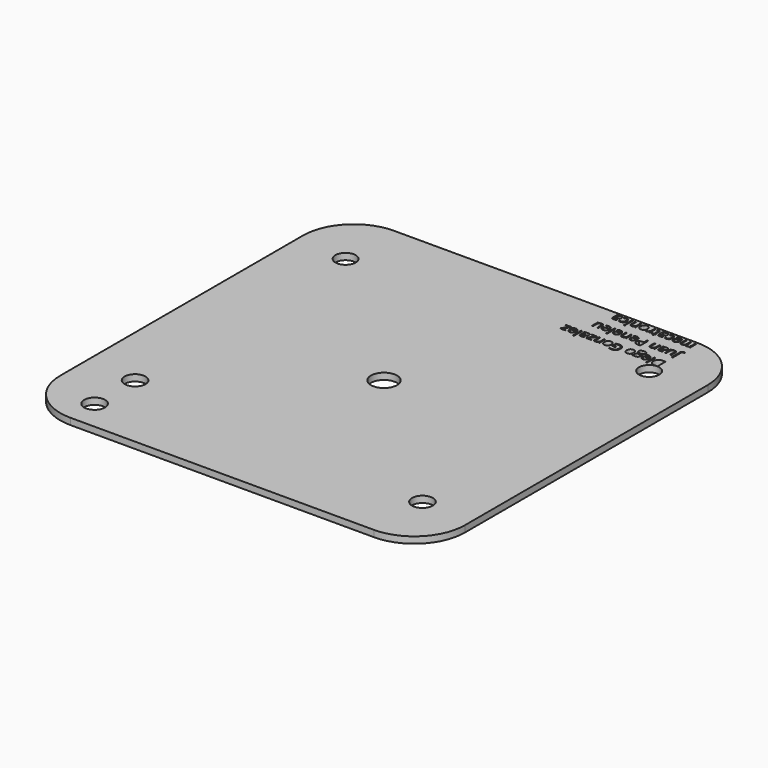
from build123d import *

# Parameters (mm, degrees)
F0_R     = 5.15
F0_R_2   = 5
F0_R_3   = 6.45
F0_W     = 0.5631510417
F0_H     = 5.2766927083
F0_H_2   = 3.7163628472
F1_DEPTH = 3.2


with BuildPart() as f1:
    # F0 (on Top) → F1 (new body)
    with BuildSketch(Plane.XY):
        with BuildLine():
            Line((75, 100), (-75, 100))
            ThreePointArc((-75, 100), (-92.6776695297, 92.6776695297), (-100, 75))
            Line((-100, 75), (-100, -75))
            ThreePointArc((-100, -75), (-92.6776695297, -92.6776695297), (-75, -100))
            Line((-75, -100), (75, -100))
            ThreePointArc((75, -100), (92.6776695297, -92.6776695297), (100, -75))
            Line((100, -75), (100, 75))
            ThreePointArc((100, 75), (92.6776695297, 92.6776695297), (75, 100))
        make_face()
        with Locations((-75, -85)):
            Circle(F0_R, mode=Mode.SUBTRACT)
        with Locations((-75, -60)):
            Circle(F0_R, mode=Mode.SUBTRACT)
        with Locations((75, -70)):
            Circle(F0_R, mode=Mode.SUBTRACT)
        with Locations((-75, 70)):
            Circle(F0_R_2, mode=Mode.SUBTRACT)
        Circle(F0_R_3, mode=Mode.SUBTRACT)
        Polygon((25.9928385417, 79.5627170139), (25.9928385417, 80), (28.6892361111, 80), (28.6892361111, 79.6169704861), (26.6612413194, 76.7209201389), (28.5633680556, 76.7209201389), (28.5633680556, 76.2836371528), (26.0438368056, 76.2836371528), (26.0438368056, 76.7209201389), (28.0447048611, 79.5627170139), align=None, mode=Mode.SUBTRACT)
        with BuildLine():
            add(Edge.make_bspline(
                [(30.0542534722, 80.0119357639), (30.3200954861, 80.068359375), (30.6966145833, 80.068359375)],
                knots=[0, 0, 0, 1, 1, 1], degree=2))
            add(Edge.make_bspline(
                [(30.6966145833, 80.068359375), (31.5201822917, 80.068359375), (31.9970703125, 79.5659722222)],
                knots=[0, 0, 0, 1, 1, 1], degree=2))
            add(Edge.make_bspline(
                [(31.9970703125, 79.5659722222), (32.4739583333, 79.0635850694), (32.4739583333, 78.1727430556)],
                knots=[0, 0, 0, 1, 1, 1], degree=2))
            add(Edge.make_bspline(
                [(32.4739583333, 78.1727430556), (32.4739583333, 77.2732204861), (32.03125, 76.7442491319)],
                knots=[0, 0, 0, 1, 1, 1], degree=2))
            add(Edge.make_bspline(
                [(32.03125, 76.7442491319), (31.5885416667, 76.2152777778), (30.8420138889, 76.2152777778)],
                knots=[0, 0, 0, 1, 1, 1], degree=2))
            add(Edge.make_bspline(
                [(30.8420138889, 76.2152777778), (30.1443142361, 76.2152777778), (29.7374131944, 76.6748046875)],
                knots=[0, 0, 0, 1, 1, 1], degree=2))
            add(Edge.make_bspline(
                [(29.7374131944, 76.6748046875), (29.3305121528, 77.1343315972), (29.3305121528, 77.8873697917)],
                knots=[0, 0, 0, 1, 1, 1], degree=2))
            Line((29.3305121528, 77.8873697917), (29.3305121528, 78.2432725694))
            Line((29.3305121528, 78.2432725694), (31.8901909722, 78.2432725694))
            add(Edge.make_bspline(
                [(31.8901909722, 78.2432725694), (31.8728298611, 78.8975694444), (31.5592447917, 79.2366536458)],
                knots=[0, 0, 0, 1, 1, 1], degree=2))
            add(Edge.make_bspline(
                [(31.5592447917, 79.2366536458), (31.2456597222, 79.5757378472), (30.6759982639, 79.5757378472)],
                knots=[0, 0, 0, 1, 1, 1], degree=2))
            add(Edge.make_bspline(
                [(30.6759982639, 79.5757378472), (30.0759548611, 79.5757378472), (29.4900173611, 79.3250868056)],
                knots=[0, 0, 0, 1, 1, 1], degree=2))
            Line((29.4900173611, 79.3250868056), (29.4900173611, 79.8274739583))
            add(Edge.make_bspline(
                [(29.4900173611, 79.8274739583), (29.7884114583, 79.9555121528), (30.0542534722, 80.0119357639)],
                knots=[0, 0, 0, 1, 1, 1], degree=2))
        make_face(mode=Mode.SUBTRACT)
        with Locations((33.7418619792, 77.3616536458)):
            Rectangle(F0_W, F0_H, mode=Mode.SUBTRACT)
        with BuildLine():
            Line((35.1822916667, 80), (35.6000434028, 80))
            Line((35.6000434028, 80), (35.7118055556, 79.4704861111))
            Line((35.7118055556, 79.4704861111), (35.7389322917, 79.4704861111))
            add(Edge.make_bspline(
                [(35.7389322917, 79.4704861111), (36.0167100694, 79.8198784722), (36.2928602431, 79.9441189236)],
                knots=[0, 0, 0, 1, 1, 1], degree=2))
            add(Edge.make_bspline(
                [(36.2928602431, 79.9441189236), (36.5690104167, 80.068359375), (36.9835069444, 80.068359375)],
                knots=[0, 0, 0, 1, 1, 1], degree=2))
            add(Edge.make_bspline(
                [(36.9835069444, 80.068359375), (37.5358072917, 80.068359375), (37.8493923611, 79.7829861111)],
                knots=[0, 0, 0, 1, 1, 1], degree=2))
            add(Edge.make_bspline(
                [(37.8493923611, 79.7829861111), (38.1629774306, 79.4976128472), (38.1629774306, 78.9724392361)],
                knots=[0, 0, 0, 1, 1, 1], degree=2))
            add(Edge.make_bspline(
                [(38.1629774306, 78.9724392361), (38.1629774306, 77.8472222222), (36.3628472222, 77.79296875)],
                knots=[0, 0, 0, 1, 1, 1], degree=2))
            Line((36.3628472222, 77.79296875), (35.732421875, 77.7723524306))
            Line((35.732421875, 77.7723524306), (35.732421875, 77.5412326389))
            add(Edge.make_bspline(
                [(35.732421875, 77.5412326389), (35.732421875, 77.1039496528), (35.9201388889, 76.8956163194)],
                knots=[0, 0, 0, 1, 1, 1], degree=2))
            add(Edge.make_bspline(
                [(35.9201388889, 76.8956163194), (36.1078559028, 76.6872829861), (36.5223524306, 76.6872829861)],
                knots=[0, 0, 0, 1, 1, 1], degree=2))
            add(Edge.make_bspline(
                [(36.5223524306, 76.6872829861), (36.9867621528, 76.6872829861), (37.5726996528, 76.9715711806)],
                knots=[0, 0, 0, 1, 1, 1], degree=2))
            Line((37.5726996528, 76.9715711806), (37.7463107639, 76.5407986111))
            add(Edge.make_bspline(
                [(37.7463107639, 76.5407986111), (37.4717881944, 76.3921440972), (37.1446397569, 76.3075086806)],
                knots=[0, 0, 0, 1, 1, 1], degree=2))
            add(Edge.make_bspline(
                [(37.1446397569, 76.3075086806), (36.8174913194, 76.2228732639), (36.4876302083, 76.2228732639)],
                knots=[0, 0, 0, 1, 1, 1], degree=2))
            add(Edge.make_bspline(
                [(36.4876302083, 76.2228732639), (35.8235677083, 76.2228732639), (35.5029296875, 76.5174696181)],
                knots=[0, 0, 0, 1, 1, 1], degree=2))
            add(Edge.make_bspline(
                [(35.5029296875, 76.5174696181), (35.1822916667, 76.8120659722), (35.1822916667, 77.4631076389)],
                knots=[0, 0, 0, 1, 1, 1], degree=2))
            Line((35.1822916667, 77.4631076389), (35.1822916667, 80))
        make_face(mode=Mode.SUBTRACT)
        Polygon((38.7565104167, 79.5627170139), (38.7565104167, 80), (41.4529079861, 80), (41.4529079861, 79.6169704861), (39.4249131944, 76.7209201389), (41.3270399306, 76.7209201389), (41.3270399306, 76.2836371528), (38.8075086806, 76.2836371528), (38.8075086806, 76.7209201389), (40.8083767361, 79.5627170139), align=None, mode=Mode.SUBTRACT)
        with BuildLine():
            Line((42.2894965278, 80), (42.8526475694, 80))
            Line((42.8526475694, 80), (42.8526475694, 77.5954861111))
            add(Edge.make_bspline(
                [(42.8526475694, 77.5954861111), (42.8526475694, 77.1419270833), (43.0593532986, 76.9178602431)],
                knots=[0, 0, 0, 1, 1, 1], degree=2))
            add(Edge.make_bspline(
                [(43.0593532986, 76.9178602431), (43.2660590278, 76.6937934028), (43.7076822917, 76.6937934028)],
                knots=[0, 0, 0, 1, 1, 1], degree=2))
            add(Edge.make_bspline(
                [(43.7076822917, 76.6937934028), (44.2903645833, 76.6937934028), (44.5616319444, 77.0090060764)],
                knots=[0, 0, 0, 1, 1, 1], degree=2))
            add(Edge.make_bspline(
                [(44.5616319444, 77.0090060764), (44.8328993056, 77.32421875), (44.8328993056, 78.0501302083)],
                knots=[0, 0, 0, 1, 1, 1], degree=2))
            Line((44.8328993056, 78.0501302083), (44.8328993056, 80))
            Line((44.8328993056, 80), (45.3960503472, 80))
            Line((45.3960503472, 80), (45.3960503472, 76.2836371528))
            Line((45.3960503472, 76.2836371528), (44.9381510417, 76.2836371528))
            Line((44.9381510417, 76.2836371528), (44.8470052083, 76.7925347222))
            Line((44.8470052083, 76.7925347222), (44.8198784722, 76.7925347222))
            add(Edge.make_bspline(
                [(44.8198784722, 76.7925347222), (44.6462673611, 76.5180121528), (44.3343098958, 76.3666449653)],
                knots=[0, 0, 0, 1, 1, 1], degree=2))
            add(Edge.make_bspline(
                [(44.3343098958, 76.3666449653), (44.0223524306, 76.2152777778), (43.6393229167, 76.2152777778)],
                knots=[0, 0, 0, 1, 1, 1], degree=2))
            add(Edge.make_bspline(
                [(43.6393229167, 76.2152777778), (42.9676649306, 76.2152777778), (42.6285807292, 76.5391710069)],
                knots=[0, 0, 0, 1, 1, 1], degree=2))
            add(Edge.make_bspline(
                [(42.6285807292, 76.5391710069), (42.2894965278, 76.8630642361), (42.2894965278, 77.5759548611)],
                knots=[0, 0, 0, 1, 1, 1], degree=2))
            Line((42.2894965278, 77.5759548611), (42.2894965278, 80))
        make_face(mode=Mode.SUBTRACT)
        with BuildLine():
            add(Edge.make_bspline(
                [(46.8429904514, 76.7344835069), (46.3834635417, 77.2536892361), (46.3834635417, 78.1380208333)],
                knots=[0, 0, 0, 1, 1, 1], degree=2))
            add(Edge.make_bspline(
                [(46.3834635417, 78.1380208333), (46.3834635417, 79.0473090278), (46.8408203125, 79.5578342014)],
                knots=[0, 0, 0, 1, 1, 1], degree=2))
            add(Edge.make_bspline(
                [(46.8408203125, 79.5578342014), (47.2981770833, 80.068359375), (48.10546875, 80.068359375)],
                knots=[0, 0, 0, 1, 1, 1], degree=2))
            add(Edge.make_bspline(
                [(48.10546875, 80.068359375), (48.6046006944, 80.068359375), (48.9908854167, 79.833984375)],
                knots=[0, 0, 0, 1, 1, 1], degree=2))
            add(Edge.make_bspline(
                [(48.9908854167, 79.833984375), (49.3771701389, 79.599609375), (49.5876736111, 79.1623263889)],
                knots=[0, 0, 0, 1, 1, 1], degree=2))
            add(Edge.make_bspline(
                [(49.5876736111, 79.1623263889), (49.7981770833, 78.7250434028), (49.7981770833, 78.1380208333)],
                knots=[0, 0, 0, 1, 1, 1], degree=2))
            add(Edge.make_bspline(
                [(49.7981770833, 78.1380208333), (49.7981770833, 77.2298177083), (49.3435329861, 76.7225477431)],
                knots=[0, 0, 0, 1, 1, 1], degree=2))
            add(Edge.make_bspline(
                [(49.3435329861, 76.7225477431), (48.8888888889, 76.2152777778), (48.0815972222, 76.2152777778)],
                knots=[0, 0, 0, 1, 1, 1], degree=2))
            add(Edge.make_bspline(
                [(48.0815972222, 76.2152777778), (47.3025173611, 76.2152777778), (46.8429904514, 76.7344835069)],
                knots=[0, 0, 0, 1, 1, 1], degree=2))
        make_face(mode=Mode.SUBTRACT)
        with Locations((42.6036241319, 86.8060980903)):
            Rectangle(F0_W, F0_H, mode=Mode.SUBTRACT)
        with BuildLine():
            Line((37.2721354167, 85.7280815972), (36.7024739583, 85.7280815972))
            Line((36.7024739583, 85.7280815972), (36.7024739583, 88.1391059028))
            add(Edge.make_bspline(
                [(36.7024739583, 88.1391059028), (36.7024739583, 88.59375), (36.4957682292, 88.8172743056)],
                knots=[0, 0, 0, 1, 1, 1], degree=2))
            add(Edge.make_bspline(
                [(36.4957682292, 88.8172743056), (36.2890625, 89.0407986111), (35.8485243056, 89.0407986111)],
                knots=[0, 0, 0, 1, 1, 1], degree=2))
            add(Edge.make_bspline(
                [(35.8485243056, 89.0407986111), (35.2647569444, 89.0407986111), (34.9956597222, 88.7223307292)],
                knots=[0, 0, 0, 1, 1, 1], degree=2))
            add(Edge.make_bspline(
                [(34.9956597222, 88.7223307292), (34.7265625, 88.4038628472), (34.7265625, 87.6812065972)],
                knots=[0, 0, 0, 1, 1, 1], degree=2))
            Line((34.7265625, 87.6812065972), (34.7265625, 85.7280815972))
            Line((34.7265625, 85.7280815972), (34.1634114583, 85.7280815972))
            Line((34.1634114583, 85.7280815972), (34.1634114583, 89.4444444444))
            Line((34.1634114583, 89.4444444444), (34.6278211806, 89.4444444444))
            Line((34.6278211806, 89.4444444444), (34.7092013889, 88.9463975694))
            Line((34.7092013889, 88.9463975694), (34.7395833333, 88.9463975694))
            add(Edge.make_bspline(
                [(34.7395833333, 88.9463975694), (34.912109375, 89.2209201389), (35.2191840278, 89.3668619792)],
                knots=[0, 0, 0, 1, 1, 1], degree=2))
            add(Edge.make_bspline(
                [(35.2191840278, 89.3668619792), (35.5262586806, 89.5128038194), (35.9201388889, 89.5128038194)],
                knots=[0, 0, 0, 1, 1, 1], degree=2))
            add(Edge.make_bspline(
                [(35.9201388889, 89.5128038194), (36.5983072917, 89.5128038194), (36.9352213542, 89.1905381944)],
                knots=[0, 0, 0, 1, 1, 1], degree=2))
            add(Edge.make_bspline(
                [(36.9352213542, 89.1905381944), (37.2721354167, 88.8682725694), (37.2721354167, 88.1597222222)],
                knots=[0, 0, 0, 1, 1, 1], degree=2))
            Line((37.2721354167, 88.1597222222), (37.2721354167, 85.7280815972))
        make_face(mode=Mode.SUBTRACT)
        with BuildLine():
            add(Edge.make_bspline(
                [(38.916015625, 89.4563802083), (39.1818576389, 89.5128038194), (39.5583767361, 89.5128038194)],
                knots=[0, 0, 0, 1, 1, 1], degree=2))
            add(Edge.make_bspline(
                [(39.5583767361, 89.5128038194), (40.3819444444, 89.5128038194), (40.8588324653, 89.0104166667)],
                knots=[0, 0, 0, 1, 1, 1], degree=2))
            add(Edge.make_bspline(
                [(40.8588324653, 89.0104166667), (41.3357204861, 88.5080295139), (41.3357204861, 87.6171875)],
                knots=[0, 0, 0, 1, 1, 1], degree=2))
            add(Edge.make_bspline(
                [(41.3357204861, 87.6171875), (41.3357204861, 86.7176649306), (40.8930121528, 86.1886935764)],
                knots=[0, 0, 0, 1, 1, 1], degree=2))
            add(Edge.make_bspline(
                [(40.8930121528, 86.1886935764), (40.4503038194, 85.6597222222), (39.7037760417, 85.6597222222)],
                knots=[0, 0, 0, 1, 1, 1], degree=2))
            add(Edge.make_bspline(
                [(39.7037760417, 85.6597222222), (39.0060763889, 85.6597222222), (38.5991753472, 86.1192491319)],
                knots=[0, 0, 0, 1, 1, 1], degree=2))
            add(Edge.make_bspline(
                [(38.5991753472, 86.1192491319), (38.1922743056, 86.5787760417), (38.1922743056, 87.3318142361)],
                knots=[0, 0, 0, 1, 1, 1], degree=2))
            Line((38.1922743056, 87.3318142361), (38.1922743056, 87.6877170139))
            Line((38.1922743056, 87.6877170139), (40.751953125, 87.6877170139))
            add(Edge.make_bspline(
                [(40.751953125, 87.6877170139), (40.7345920139, 88.3420138889), (40.4210069444, 88.6810980903)],
                knots=[0, 0, 0, 1, 1, 1], degree=2))
            add(Edge.make_bspline(
                [(40.4210069444, 88.6810980903), (40.107421875, 89.0201822917), (39.5377604167, 89.0201822917)],
                knots=[0, 0, 0, 1, 1, 1], degree=2))
            add(Edge.make_bspline(
                [(39.5377604167, 89.0201822917), (38.9377170139, 89.0201822917), (38.3517795139, 88.76953125)],
                knots=[0, 0, 0, 1, 1, 1], degree=2))
            Line((38.3517795139, 88.76953125), (38.3517795139, 89.2719184028))
            add(Edge.make_bspline(
                [(38.3517795139, 89.2719184028), (38.6501736111, 89.3999565972), (38.916015625, 89.4563802083)],
                knots=[0, 0, 0, 1, 1, 1], degree=2))
        make_face(mode=Mode.SUBTRACT)
        with BuildLine():
            add(Edge.make_bspline(
                [(44.5692274306, 89.4563802083), (44.8350694444, 89.5128038194), (45.2115885417, 89.5128038194)],
                knots=[0, 0, 0, 1, 1, 1], degree=2))
            add(Edge.make_bspline(
                [(45.2115885417, 89.5128038194), (46.03515625, 89.5128038194), (46.5120442708, 89.0104166667)],
                knots=[0, 0, 0, 1, 1, 1], degree=2))
            add(Edge.make_bspline(
                [(46.5120442708, 89.0104166667), (46.9889322917, 88.5080295139), (46.9889322917, 87.6171875)],
                knots=[0, 0, 0, 1, 1, 1], degree=2))
            add(Edge.make_bspline(
                [(46.9889322917, 87.6171875), (46.9889322917, 86.7176649306), (46.5462239583, 86.1886935764)],
                knots=[0, 0, 0, 1, 1, 1], degree=2))
            add(Edge.make_bspline(
                [(46.5462239583, 86.1886935764), (46.103515625, 85.6597222222), (45.3569878472, 85.6597222222)],
                knots=[0, 0, 0, 1, 1, 1], degree=2))
            add(Edge.make_bspline(
                [(45.3569878472, 85.6597222222), (44.6592881944, 85.6597222222), (44.2523871528, 86.1192491319)],
                knots=[0, 0, 0, 1, 1, 1], degree=2))
            add(Edge.make_bspline(
                [(44.2523871528, 86.1192491319), (43.8454861111, 86.5787760417), (43.8454861111, 87.3318142361)],
                knots=[0, 0, 0, 1, 1, 1], degree=2))
            Line((43.8454861111, 87.3318142361), (43.8454861111, 87.6877170139))
            Line((43.8454861111, 87.6877170139), (46.4051649306, 87.6877170139))
            add(Edge.make_bspline(
                [(46.4051649306, 87.6877170139), (46.3878038194, 88.3420138889), (46.07421875, 88.6810980903)],
                knots=[0, 0, 0, 1, 1, 1], degree=2))
            add(Edge.make_bspline(
                [(46.07421875, 88.6810980903), (45.7606336806, 89.0201822917), (45.1909722222, 89.0201822917)],
                knots=[0, 0, 0, 1, 1, 1], degree=2))
            add(Edge.make_bspline(
                [(45.1909722222, 89.0201822917), (44.5909288194, 89.0201822917), (44.0049913194, 88.76953125)],
                knots=[0, 0, 0, 1, 1, 1], degree=2))
            Line((44.0049913194, 88.76953125), (44.0049913194, 89.2719184028))
            add(Edge.make_bspline(
                [(44.0049913194, 89.2719184028), (44.3033854167, 89.3999565972), (44.5692274306, 89.4563802083)],
                knots=[0, 0, 0, 1, 1, 1], degree=2))
        make_face(mode=Mode.SUBTRACT)
        with BuildLine():
            Line((47.9372829861, 89.4444444444), (48.5004340278, 89.4444444444))
            Line((48.5004340278, 89.4444444444), (48.5004340278, 87.0399305556))
            add(Edge.make_bspline(
                [(48.5004340278, 87.0399305556), (48.5004340278, 86.5863715278), (48.7071397569, 86.3623046875)],
                knots=[0, 0, 0, 1, 1, 1], degree=2))
            add(Edge.make_bspline(
                [(48.7071397569, 86.3623046875), (48.9138454861, 86.1382378472), (49.35546875, 86.1382378472)],
                knots=[0, 0, 0, 1, 1, 1], degree=2))
            add(Edge.make_bspline(
                [(49.35546875, 86.1382378472), (49.9381510417, 86.1382378472), (50.2094184028, 86.4534505208)],
                knots=[0, 0, 0, 1, 1, 1], degree=2))
            add(Edge.make_bspline(
                [(50.2094184028, 86.4534505208), (50.4806857639, 86.7686631944), (50.4806857639, 87.4945746528)],
                knots=[0, 0, 0, 1, 1, 1], degree=2))
            Line((50.4806857639, 87.4945746528), (50.4806857639, 89.4444444444))
            Line((50.4806857639, 89.4444444444), (51.0438368056, 89.4444444444))
            Line((51.0438368056, 89.4444444444), (51.0438368056, 85.7280815972))
            Line((51.0438368056, 85.7280815972), (50.5859375, 85.7280815972))
            Line((50.5859375, 85.7280815972), (50.4947916667, 86.2369791667))
            Line((50.4947916667, 86.2369791667), (50.4676649306, 86.2369791667))
            add(Edge.make_bspline(
                [(50.4676649306, 86.2369791667), (50.2940538194, 85.9624565972), (49.9820963542, 85.8110894097)],
                knots=[0, 0, 0, 1, 1, 1], degree=2))
            add(Edge.make_bspline(
                [(49.9820963542, 85.8110894097), (49.6701388889, 85.6597222222), (49.287109375, 85.6597222222)],
                knots=[0, 0, 0, 1, 1, 1], degree=2))
            add(Edge.make_bspline(
                [(49.287109375, 85.6597222222), (48.6154513889, 85.6597222222), (48.2763671875, 85.9836154514)],
                knots=[0, 0, 0, 1, 1, 1], degree=2))
            add(Edge.make_bspline(
                [(48.2763671875, 85.9836154514), (47.9372829861, 86.3075086806), (47.9372829861, 87.0203993056)],
                knots=[0, 0, 0, 1, 1, 1], degree=2))
            Line((47.9372829861, 87.0203993056), (47.9372829861, 89.4444444444))
        make_face(mode=Mode.SUBTRACT)
        with BuildLine():
            add(Edge.make_bspline(
                [(43.8514539931, 94.4487847222), (43.9463975694, 94.35546875), (43.9463975694, 94.1655815972)],
                knots=[0, 0, 0, 1, 1, 1], degree=2))
            add(Edge.make_bspline(
                [(43.9463975694, 94.1655815972), (43.9463975694, 93.9724392361), (43.8514539931, 93.8823784722)],
                knots=[0, 0, 0, 1, 1, 1], degree=2))
            add(Edge.make_bspline(
                [(43.8514539931, 93.8823784722), (43.7565104167, 93.7923177083), (43.61328125, 93.7923177083)],
                knots=[0, 0, 0, 1, 1, 1], degree=2))
            add(Edge.make_bspline(
                [(43.61328125, 93.7923177083), (43.4776475694, 93.7923177083), (43.3794487847, 93.8840060764)],
                knots=[0, 0, 0, 1, 1, 1], degree=2))
            add(Edge.make_bspline(
                [(43.3794487847, 93.8840060764), (43.28125, 93.9756944444), (43.28125, 94.1655815972)],
                knots=[0, 0, 0, 1, 1, 1], degree=2))
            add(Edge.make_bspline(
                [(43.28125, 94.1655815972), (43.28125, 94.35546875), (43.3794487847, 94.4487847222)],
                knots=[0, 0, 0, 1, 1, 1], degree=2))
            add(Edge.make_bspline(
                [(43.3794487847, 94.4487847222), (43.4776475694, 94.5421006944), (43.61328125, 94.5421006944)],
                knots=[0, 0, 0, 1, 1, 1], degree=2))
            add(Edge.make_bspline(
                [(43.61328125, 94.5421006944), (43.7565104167, 94.5421006944), (43.8514539931, 94.4487847222)],
                knots=[0, 0, 0, 1, 1, 1], degree=2))
        make_face(mode=Mode.SUBTRACT)
        with BuildLine():
            Line((36.1328125, 98.8888888889), (36.5505642361, 98.8888888889))
            Line((36.5505642361, 98.8888888889), (36.6623263889, 98.359375))
            Line((36.6623263889, 98.359375), (36.689453125, 98.359375))
            add(Edge.make_bspline(
                [(36.689453125, 98.359375), (36.9672309028, 98.7087673611), (37.2433810764, 98.8330078125)],
                knots=[0, 0, 0, 1, 1, 1], degree=2))
            add(Edge.make_bspline(
                [(37.2433810764, 98.8330078125), (37.51953125, 98.9572482639), (37.9340277778, 98.9572482639)],
                knots=[0, 0, 0, 1, 1, 1], degree=2))
            add(Edge.make_bspline(
                [(37.9340277778, 98.9572482639), (38.486328125, 98.9572482639), (38.7999131944, 98.671875)],
                knots=[0, 0, 0, 1, 1, 1], degree=2))
            add(Edge.make_bspline(
                [(38.7999131944, 98.671875), (39.1134982639, 98.3865017361), (39.1134982639, 97.861328125)],
                knots=[0, 0, 0, 1, 1, 1], degree=2))
            add(Edge.make_bspline(
                [(39.1134982639, 97.861328125), (39.1134982639, 96.7361111111), (37.3133680556, 96.6818576389)],
                knots=[0, 0, 0, 1, 1, 1], degree=2))
            Line((37.3133680556, 96.6818576389), (36.6829427083, 96.6612413194))
            Line((36.6829427083, 96.6612413194), (36.6829427083, 96.4301215278))
            add(Edge.make_bspline(
                [(36.6829427083, 96.4301215278), (36.6829427083, 95.9928385417), (36.8706597222, 95.7845052083)],
                knots=[0, 0, 0, 1, 1, 1], degree=2))
            add(Edge.make_bspline(
                [(36.8706597222, 95.7845052083), (37.0583767361, 95.576171875), (37.4728732639, 95.576171875)],
                knots=[0, 0, 0, 1, 1, 1], degree=2))
            add(Edge.make_bspline(
                [(37.4728732639, 95.576171875), (37.9372829861, 95.576171875), (38.5232204861, 95.8604600694)],
                knots=[0, 0, 0, 1, 1, 1], degree=2))
            Line((38.5232204861, 95.8604600694), (38.6968315972, 95.4296875))
            add(Edge.make_bspline(
                [(38.6968315972, 95.4296875), (38.4223090278, 95.2810329861), (38.0951605903, 95.1963975694)],
                knots=[0, 0, 0, 1, 1, 1], degree=2))
            add(Edge.make_bspline(
                [(38.0951605903, 95.1963975694), (37.7680121528, 95.1117621528), (37.4381510417, 95.1117621528)],
                knots=[0, 0, 0, 1, 1, 1], degree=2))
            add(Edge.make_bspline(
                [(37.4381510417, 95.1117621528), (36.7740885417, 95.1117621528), (36.4534505208, 95.4063585069)],
                knots=[0, 0, 0, 1, 1, 1], degree=2))
            add(Edge.make_bspline(
                [(36.4534505208, 95.4063585069), (36.1328125, 95.7009548611), (36.1328125, 96.3519965278)],
                knots=[0, 0, 0, 1, 1, 1], degree=2))
            Line((36.1328125, 96.3519965278), (36.1328125, 98.8888888889))
        make_face(mode=Mode.SUBTRACT)
        with BuildLine():
            add(Edge.make_bspline(
                [(39.7178819444, 98.7630208333), (40.0900607639, 98.9572482639), (40.6564670139, 98.9572482639)],
                knots=[0, 0, 0, 1, 1, 1], degree=2))
            add(Edge.make_bspline(
                [(40.6564670139, 98.9572482639), (41.4637586806, 98.9572482639), (41.9064670139, 98.4602864583)],
                knots=[0, 0, 0, 1, 1, 1], degree=2))
            add(Edge.make_bspline(
                [(41.9064670139, 98.4602864583), (42.3491753472, 97.9633246528), (42.3491753472, 97.0540364583)],
                knots=[0, 0, 0, 1, 1, 1], degree=2))
            add(Edge.make_bspline(
                [(42.3491753472, 97.0540364583), (42.3491753472, 96.1219618056), (41.8994140625, 95.6130642361)],
                knots=[0, 0, 0, 1, 1, 1], degree=2))
            add(Edge.make_bspline(
                [(41.8994140625, 95.6130642361), (41.4496527778, 95.1041666667), (40.6195746528, 95.1041666667)],
                knots=[0, 0, 0, 1, 1, 1], degree=2))
            add(Edge.make_bspline(
                [(40.6195746528, 95.1041666667), (40.3515625, 95.1041666667), (40.0835503472, 95.1622178819)],
                knots=[0, 0, 0, 1, 1, 1], degree=2))
            add(Edge.make_bspline(
                [(40.0835503472, 95.1622178819), (39.8155381944, 95.2202690972), (39.6636284722, 95.2983940972)],
                knots=[0, 0, 0, 1, 1, 1], degree=2))
            Line((39.6636284722, 95.2983940972), (39.8361545139, 95.7758246528))
            add(Edge.make_bspline(
                [(39.8361545139, 95.7758246528), (40.0227864583, 95.7009548611), (40.2430555556, 95.6521267361)],
                knots=[0, 0, 0, 1, 1, 1], degree=2))
            add(Edge.make_bspline(
                [(40.2430555556, 95.6521267361), (40.4633246528, 95.6032986111), (40.6325954861, 95.6032986111)],
                knots=[0, 0, 0, 1, 1, 1], degree=2))
            add(Edge.make_bspline(
                [(40.6325954861, 95.6032986111), (41.7654079861, 95.6032986111), (41.7654079861, 97.0475260417)],
                knots=[0, 0, 0, 1, 1, 1], degree=2))
            add(Edge.make_bspline(
                [(41.7654079861, 97.0475260417), (41.7654079861, 97.7322048611), (41.4892578125, 98.0984157986)],
                knots=[0, 0, 0, 1, 1, 1], degree=2))
            add(Edge.make_bspline(
                [(41.4892578125, 98.0984157986), (41.2131076389, 98.4646267361), (40.6705729167, 98.4646267361)],
                knots=[0, 0, 0, 1, 1, 1], degree=2))
            add(Edge.make_bspline(
                [(40.6705729167, 98.4646267361), (40.2061631944, 98.4646267361), (39.7178819444, 98.2649739583)],
                knots=[0, 0, 0, 1, 1, 1], degree=2))
            Line((39.7178819444, 98.2649739583), (39.7178819444, 98.7630208333))
        make_face(mode=Mode.SUBTRACT)
        with Locations((43.6170789931, 97.0307074653)):
            Rectangle(F0_W, F0_H_2, mode=Mode.SUBTRACT)
        with BuildLine():
            Line((45.0542534722, 98.8888888889), (45.6174045139, 98.8888888889))
            Line((45.6174045139, 98.8888888889), (45.6174045139, 96.484375))
            add(Edge.make_bspline(
                [(45.6174045139, 96.484375), (45.6174045139, 96.0308159722), (45.8241102431, 95.8067491319)],
                knots=[0, 0, 0, 1, 1, 1], degree=2))
            add(Edge.make_bspline(
                [(45.8241102431, 95.8067491319), (46.0308159722, 95.5826822917), (46.4724392361, 95.5826822917)],
                knots=[0, 0, 0, 1, 1, 1], degree=2))
            add(Edge.make_bspline(
                [(46.4724392361, 95.5826822917), (47.0551215278, 95.5826822917), (47.3263888889, 95.8978949653)],
                knots=[0, 0, 0, 1, 1, 1], degree=2))
            add(Edge.make_bspline(
                [(47.3263888889, 95.8978949653), (47.59765625, 96.2131076389), (47.59765625, 96.9390190972)],
                knots=[0, 0, 0, 1, 1, 1], degree=2))
            Line((47.59765625, 96.9390190972), (47.59765625, 98.8888888889))
            Line((47.59765625, 98.8888888889), (48.1608072917, 98.8888888889))
            Line((48.1608072917, 98.8888888889), (48.1608072917, 95.1725260417))
            Line((48.1608072917, 95.1725260417), (47.7029079861, 95.1725260417))
            Line((47.7029079861, 95.1725260417), (47.6117621528, 95.6814236111))
            Line((47.6117621528, 95.6814236111), (47.5846354167, 95.6814236111))
            add(Edge.make_bspline(
                [(47.5846354167, 95.6814236111), (47.4110243056, 95.4069010417), (47.0990668403, 95.2555338542)],
                knots=[0, 0, 0, 1, 1, 1], degree=2))
            add(Edge.make_bspline(
                [(47.0990668403, 95.2555338542), (46.787109375, 95.1041666667), (46.4040798611, 95.1041666667)],
                knots=[0, 0, 0, 1, 1, 1], degree=2))
            add(Edge.make_bspline(
                [(46.4040798611, 95.1041666667), (45.732421875, 95.1041666667), (45.3933376736, 95.4280598958)],
                knots=[0, 0, 0, 1, 1, 1], degree=2))
            add(Edge.make_bspline(
                [(45.3933376736, 95.4280598958), (45.0542534722, 95.751953125), (45.0542534722, 96.46484375)],
                knots=[0, 0, 0, 1, 1, 1], degree=2))
            Line((45.0542534722, 96.46484375), (45.0542534722, 98.8888888889))
        make_face(mode=Mode.SUBTRACT)
        with Locations((75, 70)):
            Circle(F0_R_2, mode=Mode.SUBTRACT)
        with BuildLine():
            Line((52.3806423611, 77.9177517361), (52.3806423611, 77.40234375))
            Line((52.3806423611, 77.40234375), (50.6955295139, 77.40234375))
            Line((50.6955295139, 77.40234375), (50.6955295139, 79.8133680556))
            add(Edge.make_bspline(
                [(50.6955295139, 79.8133680556), (51.0894097222, 79.9392361111), (51.4963107639, 80.0037977431)],
                knots=[0, 0, 0, 1, 1, 1], degree=2))
            add(Edge.make_bspline(
                [(51.4963107639, 80.0037977431), (51.9032118056, 80.068359375), (52.4392361111, 80.068359375)],
                knots=[0, 0, 0, 1, 1, 1], degree=2))
            add(Edge.make_bspline(
                [(52.4392361111, 80.068359375), (53.564453125, 80.068359375), (54.1916232639, 79.3983289931)],
                knots=[0, 0, 0, 1, 1, 1], degree=2))
            add(Edge.make_bspline(
                [(54.1916232639, 79.3983289931), (54.8187934028, 78.7282986111), (54.8187934028, 77.5217013889)],
                knots=[0, 0, 0, 1, 1, 1], degree=2))
            add(Edge.make_bspline(
                [(54.8187934028, 77.5217013889), (54.8187934028, 76.748046875), (54.5084635417, 76.1664496528)],
                knots=[0, 0, 0, 1, 1, 1], degree=2))
            add(Edge.make_bspline(
                [(54.5084635417, 76.1664496528), (54.1981336806, 75.5848524306), (53.6149088542, 75.2783203125)],
                knots=[0, 0, 0, 1, 1, 1], degree=2))
            add(Edge.make_bspline(
                [(53.6149088542, 75.2783203125), (53.0316840278, 74.9717881944), (52.2493489583, 74.9717881944)],
                knots=[0, 0, 0, 1, 1, 1], degree=2))
            add(Edge.make_bspline(
                [(52.2493489583, 74.9717881944), (51.455078125, 74.9717881944), (50.7703993056, 75.2625868056)],
                knots=[0, 0, 0, 1, 1, 1], degree=2))
            Line((50.7703993056, 75.2625868056), (50.9939236111, 75.771484375))
            add(Edge.make_bspline(
                [(50.9939236111, 75.771484375), (51.6655815972, 75.4871961806), (52.2862413194, 75.4871961806)],
                knots=[0, 0, 0, 1, 1, 1], degree=2))
            add(Edge.make_bspline(
                [(52.2862413194, 75.4871961806), (53.1911892361, 75.4871961806), (53.7000868056, 76.0259331597)],
                knots=[0, 0, 0, 1, 1, 1], degree=2))
            add(Edge.make_bspline(
                [(53.7000868056, 76.0259331597), (54.208984375, 76.5646701389), (54.208984375, 77.5217013889)],
                knots=[0, 0, 0, 1, 1, 1], degree=2))
            add(Edge.make_bspline(
                [(54.208984375, 77.5217013889), (54.208984375, 78.525390625), (53.7190755208, 79.0440538194)],
                knots=[0, 0, 0, 1, 1, 1], degree=2))
            add(Edge.make_bspline(
                [(53.7190755208, 79.0440538194), (53.2291666667, 79.5627170139), (52.2797309028, 79.5627170139)],
                knots=[0, 0, 0, 1, 1, 1], degree=2))
            add(Edge.make_bspline(
                [(52.2797309028, 79.5627170139), (51.7643229167, 79.5627170139), (51.2727864583, 79.443359375)],
                knots=[0, 0, 0, 1, 1, 1], degree=2))
            Line((51.2727864583, 79.443359375), (51.2727864583, 77.9177517361))
            Line((51.2727864583, 77.9177517361), (52.3806423611, 77.9177517361))
        make_face(mode=Mode.SUBTRACT)
        with BuildLine():
            add(Edge.make_bspline(
                [(57.8976779514, 76.7344835069), (57.4381510417, 77.2536892361), (57.4381510417, 78.1380208333)],
                knots=[0, 0, 0, 1, 1, 1], degree=2))
            add(Edge.make_bspline(
                [(57.4381510417, 78.1380208333), (57.4381510417, 79.0473090278), (57.8955078125, 79.5578342014)],
                knots=[0, 0, 0, 1, 1, 1], degree=2))
            add(Edge.make_bspline(
                [(57.8955078125, 79.5578342014), (58.3528645833, 80.068359375), (59.16015625, 80.068359375)],
                knots=[0, 0, 0, 1, 1, 1], degree=2))
            add(Edge.make_bspline(
                [(59.16015625, 80.068359375), (59.6592881944, 80.068359375), (60.0455729167, 79.833984375)],
                knots=[0, 0, 0, 1, 1, 1], degree=2))
            add(Edge.make_bspline(
                [(60.0455729167, 79.833984375), (60.4318576389, 79.599609375), (60.6423611111, 79.1623263889)],
                knots=[0, 0, 0, 1, 1, 1], degree=2))
            add(Edge.make_bspline(
                [(60.6423611111, 79.1623263889), (60.8528645833, 78.7250434028), (60.8528645833, 78.1380208333)],
                knots=[0, 0, 0, 1, 1, 1], degree=2))
            add(Edge.make_bspline(
                [(60.8528645833, 78.1380208333), (60.8528645833, 77.2298177083), (60.3982204861, 76.7225477431)],
                knots=[0, 0, 0, 1, 1, 1], degree=2))
            add(Edge.make_bspline(
                [(60.3982204861, 76.7225477431), (59.9435763889, 76.2152777778), (59.1362847222, 76.2152777778)],
                knots=[0, 0, 0, 1, 1, 1], degree=2))
            add(Edge.make_bspline(
                [(59.1362847222, 76.2152777778), (58.3572048611, 76.2152777778), (57.8976779514, 76.7344835069)],
                knots=[0, 0, 0, 1, 1, 1], degree=2))
        make_face(mode=Mode.SUBTRACT)
        with BuildLine():
            add(Edge.make_bspline(
                [(57.7506510417, 84.4867621528), (55.8930121528, 84.4867621528), (55.8930121528, 85.9309895833)],
                knots=[0, 0, 0, 1, 1, 1], degree=2))
            add(Edge.make_bspline(
                [(55.8930121528, 85.9309895833), (55.8930121528, 86.6840277778), (56.4067925347, 87.0893012153)],
                knots=[0, 0, 0, 1, 1, 1], degree=2))
            add(Edge.make_bspline(
                [(56.4067925347, 87.0893012153), (56.9205729167, 87.4945746528), (57.8765190972, 87.4945746528)],
                knots=[0, 0, 0, 1, 1, 1], degree=2))
            Line((57.8765190972, 87.4945746528), (58.4602864583, 87.4945746528))
            Line((58.4602864583, 87.4945746528), (58.4602864583, 89.4444444444))
            Line((58.4602864583, 89.4444444444), (59.0364583333, 89.4444444444))
            Line((59.0364583333, 89.4444444444), (59.0364583333, 84.4867621528))
            Line((59.0364583333, 84.4867621528), (57.7506510417, 84.4867621528))
        make_face(mode=Mode.SUBTRACT)
        with BuildLine():
            Line((62.6931423611, 76.2836371528), (61.4084201389, 76.2836371528))
            Line((61.4084201389, 76.2836371528), (61.4084201389, 76.6395399306))
            Line((61.4084201389, 76.6395399306), (62.0963541667, 76.7209201389))
            add(Edge.make_bspline(
                [(62.0963541667, 76.7209201389), (62.001953125, 76.8391927083), (61.9270833333, 77.03125)],
                knots=[0, 0, 0, 1, 1, 1], degree=2))
            add(Edge.make_bspline(
                [(61.9270833333, 77.03125), (61.8522135417, 77.2233072917), (61.8522135417, 77.4631076389)],
                knots=[0, 0, 0, 1, 1, 1], degree=2))
            add(Edge.make_bspline(
                [(61.8522135417, 77.4631076389), (61.8522135417, 78.0099826389), (62.2254774306, 78.3355034722)],
                knots=[0, 0, 0, 1, 1, 1], degree=2))
            add(Edge.make_bspline(
                [(62.2254774306, 78.3355034722), (62.5987413194, 78.6610243056), (63.2497829861, 78.6610243056)],
                knots=[0, 0, 0, 1, 1, 1], degree=2))
            add(Edge.make_bspline(
                [(63.2497829861, 78.6610243056), (63.4157986111, 78.6610243056), (63.5611979167, 78.6338975694)],
                knots=[0, 0, 0, 1, 1, 1], degree=2))
            add(Edge.make_bspline(
                [(63.5611979167, 78.6338975694), (63.9203559028, 78.8237847222), (63.9203559028, 79.111328125)],
                knots=[0, 0, 0, 1, 1, 1], degree=2))
            add(Edge.make_bspline(
                [(63.9203559028, 79.111328125), (63.9203559028, 79.2643229167), (63.7950303819, 79.3370225694)],
                knots=[0, 0, 0, 1, 1, 1], degree=2))
            add(Edge.make_bspline(
                [(63.7950303819, 79.3370225694), (63.6697048611, 79.4097222222), (63.3648003472, 79.4097222222)],
                knots=[0, 0, 0, 1, 1, 1], degree=2))
            Line((63.3648003472, 79.4097222222), (62.7072482639, 79.4097222222))
            add(Edge.make_bspline(
                [(62.7072482639, 79.4097222222), (62.1028645833, 79.4097222222), (61.7795138889, 79.6641710069)],
                knots=[0, 0, 0, 1, 1, 1], degree=2))
            add(Edge.make_bspline(
                [(61.7795138889, 79.6641710069), (61.4561631944, 79.9186197917), (61.4561631944, 80.4036458333)],
                knots=[0, 0, 0, 1, 1, 1], degree=2))
            add(Edge.make_bspline(
                [(61.4561631944, 80.4036458333), (61.4561631944, 81.0210503472), (61.9509548611, 81.3449435764)],
                knots=[0, 0, 0, 1, 1, 1], degree=2))
            add(Edge.make_bspline(
                [(61.9509548611, 81.3449435764), (62.4457465278, 81.6688368056), (63.3951822917, 81.6688368056)],
                knots=[0, 0, 0, 1, 1, 1], degree=2))
            add(Edge.make_bspline(
                [(63.3951822917, 81.6688368056), (64.1243489583, 81.6688368056), (64.5193142361, 81.3975694444)],
                knots=[0, 0, 0, 1, 1, 1], degree=2))
            add(Edge.make_bspline(
                [(64.5193142361, 81.3975694444), (64.9142795139, 81.1263020833), (64.9142795139, 80.6304253472)],
                knots=[0, 0, 0, 1, 1, 1], degree=2))
            add(Edge.make_bspline(
                [(64.9142795139, 80.6304253472), (64.9142795139, 80.2918836806), (64.697265625, 80.0439453125)],
                knots=[0, 0, 0, 1, 1, 1], degree=2))
            add(Edge.make_bspline(
                [(64.697265625, 80.0439453125), (64.4802517361, 79.7960069444), (64.0874565972, 79.7081163194)],
                knots=[0, 0, 0, 1, 1, 1], degree=2))
            add(Edge.make_bspline(
                [(64.0874565972, 79.7081163194), (64.2296006944, 79.6440972222), (64.326171875, 79.5084635417)],
                knots=[0, 0, 0, 1, 1, 1], degree=2))
            add(Edge.make_bspline(
                [(64.326171875, 79.5084635417), (64.4227430556, 79.3728298611), (64.4227430556, 79.1927083333)],
                knots=[0, 0, 0, 1, 1, 1], degree=2))
            add(Edge.make_bspline(
                [(64.4227430556, 79.1927083333), (64.4227430556, 78.9898003472), (64.3142361111, 78.8368055556)],
                knots=[0, 0, 0, 1, 1, 1], degree=2))
            add(Edge.make_bspline(
                [(64.3142361111, 78.8368055556), (64.2057291667, 78.6838107639), (63.9713541667, 78.5416666667)],
                knots=[0, 0, 0, 1, 1, 1], degree=2))
            add(Edge.make_bspline(
                [(63.9713541667, 78.5416666667), (64.2599826389, 78.4233940972), (64.4411892361, 78.1385633681)],
                knots=[0, 0, 0, 1, 1, 1], degree=2))
            add(Edge.make_bspline(
                [(64.4411892361, 78.1385633681), (64.6223958333, 77.8537326389), (64.6223958333, 77.4869791667)],
                knots=[0, 0, 0, 1, 1, 1], degree=2))
            add(Edge.make_bspline(
                [(64.6223958333, 77.4869791667), (64.6223958333, 76.8771701389), (64.2561848958, 76.5462239583)],
                knots=[0, 0, 0, 1, 1, 1], degree=2))
            add(Edge.make_bspline(
                [(64.2561848958, 76.5462239583), (63.8899739583, 76.2152777778), (63.2194010417, 76.2152777778)],
                knots=[0, 0, 0, 1, 1, 1], degree=2))
            add(Edge.make_bspline(
                [(63.2194010417, 76.2152777778), (62.9275173611, 76.2152777778), (62.6931423611, 76.2836371528)],
                knots=[0, 0, 0, 1, 1, 1], degree=2))
        make_face(mode=Mode.SUBTRACT)
        with BuildLine():
            add(Edge.make_bspline(
                [(66.1338975694, 80.0119357639), (66.3997395833, 80.068359375), (66.7762586806, 80.068359375)],
                knots=[0, 0, 0, 1, 1, 1], degree=2))
            add(Edge.make_bspline(
                [(66.7762586806, 80.068359375), (67.5998263889, 80.068359375), (68.0767144097, 79.5659722222)],
                knots=[0, 0, 0, 1, 1, 1], degree=2))
            add(Edge.make_bspline(
                [(68.0767144097, 79.5659722222), (68.5536024306, 79.0635850694), (68.5536024306, 78.1727430556)],
                knots=[0, 0, 0, 1, 1, 1], degree=2))
            add(Edge.make_bspline(
                [(68.5536024306, 78.1727430556), (68.5536024306, 77.2732204861), (68.1108940972, 76.7442491319)],
                knots=[0, 0, 0, 1, 1, 1], degree=2))
            add(Edge.make_bspline(
                [(68.1108940972, 76.7442491319), (67.6681857639, 76.2152777778), (66.9216579861, 76.2152777778)],
                knots=[0, 0, 0, 1, 1, 1], degree=2))
            add(Edge.make_bspline(
                [(66.9216579861, 76.2152777778), (66.2239583333, 76.2152777778), (65.8170572917, 76.6748046875)],
                knots=[0, 0, 0, 1, 1, 1], degree=2))
            add(Edge.make_bspline(
                [(65.8170572917, 76.6748046875), (65.41015625, 77.1343315972), (65.41015625, 77.8873697917)],
                knots=[0, 0, 0, 1, 1, 1], degree=2))
            Line((65.41015625, 77.8873697917), (65.41015625, 78.2432725694))
            Line((65.41015625, 78.2432725694), (67.9698350694, 78.2432725694))
            add(Edge.make_bspline(
                [(67.9698350694, 78.2432725694), (67.9524739583, 78.8975694444), (67.6388888889, 79.2366536458)],
                knots=[0, 0, 0, 1, 1, 1], degree=2))
            add(Edge.make_bspline(
                [(67.6388888889, 79.2366536458), (67.3253038194, 79.5757378472), (66.7556423611, 79.5757378472)],
                knots=[0, 0, 0, 1, 1, 1], degree=2))
            add(Edge.make_bspline(
                [(66.7556423611, 79.5757378472), (66.1555989583, 79.5757378472), (65.5696614583, 79.3250868056)],
                knots=[0, 0, 0, 1, 1, 1], degree=2))
            Line((65.5696614583, 79.3250868056), (65.5696614583, 79.8274739583))
            add(Edge.make_bspline(
                [(65.5696614583, 79.8274739583), (65.8680555556, 79.9555121528), (66.1338975694, 80.0119357639)],
                knots=[0, 0, 0, 1, 1, 1], degree=2))
        make_face(mode=Mode.SUBTRACT)
        with BuildLine():
            add(Edge.make_bspline(
                [(70.0558810764, 75.5598958333), (70.1508246528, 75.4665798611), (70.1508246528, 75.2766927083)],
                knots=[0, 0, 0, 1, 1, 1], degree=2))
            add(Edge.make_bspline(
                [(70.1508246528, 75.2766927083), (70.1508246528, 75.0835503472), (70.0558810764, 74.9934895833)],
                knots=[0, 0, 0, 1, 1, 1], degree=2))
            add(Edge.make_bspline(
                [(70.0558810764, 74.9934895833), (69.9609375, 74.9034288194), (69.8177083333, 74.9034288194)],
                knots=[0, 0, 0, 1, 1, 1], degree=2))
            add(Edge.make_bspline(
                [(69.8177083333, 74.9034288194), (69.6820746528, 74.9034288194), (69.5838758681, 74.9951171875)],
                knots=[0, 0, 0, 1, 1, 1], degree=2))
            add(Edge.make_bspline(
                [(69.5838758681, 74.9951171875), (69.4856770833, 75.0868055556), (69.4856770833, 75.2766927083)],
                knots=[0, 0, 0, 1, 1, 1], degree=2))
            add(Edge.make_bspline(
                [(69.4856770833, 75.2766927083), (69.4856770833, 75.4665798611), (69.5838758681, 75.5598958333)],
                knots=[0, 0, 0, 1, 1, 1], degree=2))
            add(Edge.make_bspline(
                [(69.5838758681, 75.5598958333), (69.6820746528, 75.6532118056), (69.8177083333, 75.6532118056)],
                knots=[0, 0, 0, 1, 1, 1], degree=2))
            add(Edge.make_bspline(
                [(69.8177083333, 75.6532118056), (69.9609375, 75.6532118056), (70.0558810764, 75.5598958333)],
                knots=[0, 0, 0, 1, 1, 1], degree=2))
        make_face(mode=Mode.SUBTRACT)
        with BuildLine():
            add(Edge.make_bspline(
                [(71.7648654514, 75.6830512153), (71.1241319444, 76.3237847222), (71.1241319444, 77.4739583333)],
                knots=[0, 0, 0, 1, 1, 1], degree=2))
            add(Edge.make_bspline(
                [(71.1241319444, 77.4739583333), (71.1241319444, 78.701171875), (71.7903645833, 79.3505859375)],
                knots=[0, 0, 0, 1, 1, 1], degree=2))
            add(Edge.make_bspline(
                [(71.7903645833, 79.3505859375), (72.4565972222, 80), (73.7076822917, 80)],
                knots=[0, 0, 0, 1, 1, 1], degree=2))
            Line((73.7076822917, 80), (75.0813802083, 80))
            Line((75.0813802083, 80), (75.0813802083, 75.0423177083))
            Line((75.0813802083, 75.0423177083), (73.5622829861, 75.0423177083))
            add(Edge.make_bspline(
                [(73.5622829861, 75.0423177083), (72.4055989583, 75.0423177083), (71.7648654514, 75.6830512153)],
                knots=[0, 0, 0, 1, 1, 1], degree=2))
        make_face(mode=Mode.SUBTRACT)
        with Locations((69.8215060764, 78.1418185764)):
            Rectangle(F0_W, F0_H_2, mode=Mode.SUBTRACT)
        with BuildLine():
            add(Edge.make_bspline(
                [(52.7278645833, 89.4563802083), (52.9937065972, 89.5128038194), (53.3702256944, 89.5128038194)],
                knots=[0, 0, 0, 1, 1, 1], degree=2))
            add(Edge.make_bspline(
                [(53.3702256944, 89.5128038194), (54.1937934028, 89.5128038194), (54.6706814236, 89.0104166667)],
                knots=[0, 0, 0, 1, 1, 1], degree=2))
            add(Edge.make_bspline(
                [(54.6706814236, 89.0104166667), (55.1475694444, 88.5080295139), (55.1475694444, 87.6171875)],
                knots=[0, 0, 0, 1, 1, 1], degree=2))
            add(Edge.make_bspline(
                [(55.1475694444, 87.6171875), (55.1475694444, 86.7176649306), (54.7048611111, 86.1886935764)],
                knots=[0, 0, 0, 1, 1, 1], degree=2))
            add(Edge.make_bspline(
                [(54.7048611111, 86.1886935764), (54.2621527778, 85.6597222222), (53.515625, 85.6597222222)],
                knots=[0, 0, 0, 1, 1, 1], degree=2))
            add(Edge.make_bspline(
                [(53.515625, 85.6597222222), (52.8179253472, 85.6597222222), (52.4110243056, 86.1192491319)],
                knots=[0, 0, 0, 1, 1, 1], degree=2))
            add(Edge.make_bspline(
                [(52.4110243056, 86.1192491319), (52.0041232639, 86.5787760417), (52.0041232639, 87.3318142361)],
                knots=[0, 0, 0, 1, 1, 1], degree=2))
            Line((52.0041232639, 87.3318142361), (52.0041232639, 87.6877170139))
            Line((52.0041232639, 87.6877170139), (54.5638020833, 87.6877170139))
            add(Edge.make_bspline(
                [(54.5638020833, 87.6877170139), (54.5464409722, 88.3420138889), (54.2328559028, 88.6810980903)],
                knots=[0, 0, 0, 1, 1, 1], degree=2))
            add(Edge.make_bspline(
                [(54.2328559028, 88.6810980903), (53.9192708333, 89.0201822917), (53.349609375, 89.0201822917)],
                knots=[0, 0, 0, 1, 1, 1], degree=2))
            add(Edge.make_bspline(
                [(53.349609375, 89.0201822917), (52.7495659722, 89.0201822917), (52.1636284722, 88.76953125)],
                knots=[0, 0, 0, 1, 1, 1], degree=2))
            Line((52.1636284722, 88.76953125), (52.1636284722, 89.2719184028))
            add(Edge.make_bspline(
                [(52.1636284722, 89.2719184028), (52.4620225694, 89.3999565972), (52.7278645833, 89.4563802083)],
                knots=[0, 0, 0, 1, 1, 1], degree=2))
        make_face(mode=Mode.SUBTRACT)
        with BuildLine():
            add(Edge.make_bspline(
                [(49.6077473958, 95.6233723958), (49.1482204861, 96.142578125), (49.1482204861, 97.0269097222)],
                knots=[0, 0, 0, 1, 1, 1], degree=2))
            add(Edge.make_bspline(
                [(49.1482204861, 97.0269097222), (49.1482204861, 97.9361979167), (49.6055772569, 98.4467230903)],
                knots=[0, 0, 0, 1, 1, 1], degree=2))
            add(Edge.make_bspline(
                [(49.6055772569, 98.4467230903), (50.0629340278, 98.9572482639), (50.8702256944, 98.9572482639)],
                knots=[0, 0, 0, 1, 1, 1], degree=2))
            add(Edge.make_bspline(
                [(50.8702256944, 98.9572482639), (51.3693576389, 98.9572482639), (51.7556423611, 98.7228732639)],
                knots=[0, 0, 0, 1, 1, 1], degree=2))
            add(Edge.make_bspline(
                [(51.7556423611, 98.7228732639), (52.1419270833, 98.4884982639), (52.3524305556, 98.0512152778)],
                knots=[0, 0, 0, 1, 1, 1], degree=2))
            add(Edge.make_bspline(
                [(52.3524305556, 98.0512152778), (52.5629340278, 97.6139322917), (52.5629340278, 97.0269097222)],
                knots=[0, 0, 0, 1, 1, 1], degree=2))
            add(Edge.make_bspline(
                [(52.5629340278, 97.0269097222), (52.5629340278, 96.1187065972), (52.1082899306, 95.6114366319)],
                knots=[0, 0, 0, 1, 1, 1], degree=2))
            add(Edge.make_bspline(
                [(52.1082899306, 95.6114366319), (51.6536458333, 95.1041666667), (50.8463541667, 95.1041666667)],
                knots=[0, 0, 0, 1, 1, 1], degree=2))
            add(Edge.make_bspline(
                [(50.8463541667, 95.1041666667), (50.0672743056, 95.1041666667), (49.6077473958, 95.6233723958)],
                knots=[0, 0, 0, 1, 1, 1], degree=2))
        make_face(mode=Mode.SUBTRACT)
        with BuildLine():
            add(Edge.make_bspline(
                [(54.1362847222, 95.3011067708), (53.8444010417, 95.1041666667), (53.4950086806, 95.1041666667)],
                knots=[0, 0, 0, 1, 1, 1], degree=2))
            add(Edge.make_bspline(
                [(53.4950086806, 95.1041666667), (53.2476128472, 95.1041666667), (53.0512152778, 95.1453993056)],
                knots=[0, 0, 0, 1, 1, 1], degree=2))
            Line((53.0512152778, 95.1453993056), (53.1293402778, 95.6673177083))
            add(Edge.make_bspline(
                [(53.1293402778, 95.6673177083), (53.359375, 95.6163194444), (53.5362413194, 95.6163194444)],
                knots=[0, 0, 0, 1, 1, 1], degree=2))
            add(Edge.make_bspline(
                [(53.5362413194, 95.6163194444), (53.9876302083, 95.6163194444), (54.3077256944, 95.9825303819)],
                knots=[0, 0, 0, 1, 1, 1], degree=2))
            add(Edge.make_bspline(
                [(54.3077256944, 95.9825303819), (54.6278211806, 96.3487413194), (54.6278211806, 96.89453125)],
                knots=[0, 0, 0, 1, 1, 1], degree=2))
            Line((54.6278211806, 96.89453125), (54.6278211806, 98.8888888889))
            Line((54.6278211806, 98.8888888889), (55.1909722222, 98.8888888889))
            Line((55.1909722222, 98.8888888889), (55.1909722222, 95.1725260417))
            Line((55.1909722222, 95.1725260417), (54.7265625, 95.1725260417))
            Line((54.7265625, 95.1725260417), (54.6614583333, 95.8604600694))
            Line((54.6614583333, 95.8604600694), (54.6343315972, 95.8604600694))
            add(Edge.make_bspline(
                [(54.6343315972, 95.8604600694), (54.4281684028, 95.498046875), (54.1362847222, 95.3011067708)],
                knots=[0, 0, 0, 1, 1, 1], degree=2))
        make_face(mode=Mode.SUBTRACT)
        with BuildLine():
            add(Edge.make_bspline(
                [(56.8793402778, 98.3121744792), (56.7198350694, 98.4917534722), (56.4420572917, 98.4917534722)],
                knots=[0, 0, 0, 1, 1, 1], degree=2))
            add(Edge.make_bspline(
                [(56.4420572917, 98.4917534722), (56.2923177083, 98.4917534722), (56.1534288194, 98.4700520833)],
                knots=[0, 0, 0, 1, 1, 1], degree=2))
            add(Edge.make_bspline(
                [(56.1534288194, 98.4700520833), (56.0145399306, 98.4483506944), (55.9331597222, 98.4244791667)],
                knots=[0, 0, 0, 1, 1, 1], degree=2))
            Line((55.9331597222, 98.4244791667), (55.9331597222, 98.8552517361))
            add(Edge.make_bspline(
                [(55.9331597222, 98.8552517361), (56.0243055556, 98.8986545139), (56.2022569444, 98.9279513889)],
                knots=[0, 0, 0, 1, 1, 1], degree=2))
            add(Edge.make_bspline(
                [(56.2022569444, 98.9279513889), (56.3802083333, 98.9572482639), (56.5234375, 98.9572482639)],
                knots=[0, 0, 0, 1, 1, 1], degree=2))
            add(Edge.make_bspline(
                [(56.5234375, 98.9572482639), (57.6009114583, 98.9572482639), (57.6009114583, 97.8211805556)],
                knots=[0, 0, 0, 1, 1, 1], degree=2))
            Line((57.6009114583, 97.8211805556), (57.6009114583, 95.6098090278))
            Line((57.6009114583, 95.6098090278), (58.1336805556, 95.6098090278))
            Line((58.1336805556, 95.6098090278), (58.1336805556, 95.3385416667))
            Line((58.1336805556, 95.3385416667), (57.6009114583, 95.1041666667))
            Line((57.6009114583, 95.1041666667), (57.3643663194, 94.3109809028))
            Line((57.3643663194, 94.3109809028), (57.0388454861, 94.3109809028))
            Line((57.0388454861, 94.3109809028), (57.0388454861, 95.1725260417))
            Line((57.0388454861, 95.1725260417), (55.9602864583, 95.1725260417))
            Line((55.9602864583, 95.1725260417), (55.9602864583, 95.6098090278))
            Line((55.9602864583, 95.6098090278), (57.0388454861, 95.6098090278))
            Line((57.0388454861, 95.6098090278), (57.0388454861, 97.7973090278))
            add(Edge.make_bspline(
                [(57.0388454861, 97.7973090278), (57.0388454861, 98.1325954861), (56.8793402778, 98.3121744792)],
                knots=[0, 0, 0, 1, 1, 1], degree=2))
        make_face(mode=Mode.SUBTRACT)
        with BuildLine():
            Line((58.8009982639, 98.8888888889), (59.21875, 98.8888888889))
            Line((59.21875, 98.8888888889), (59.3305121528, 98.359375))
            Line((59.3305121528, 98.359375), (59.3576388889, 98.359375))
            add(Edge.make_bspline(
                [(59.3576388889, 98.359375), (59.6354166667, 98.7087673611), (59.9115668403, 98.8330078125)],
                knots=[0, 0, 0, 1, 1, 1], degree=2))
            add(Edge.make_bspline(
                [(59.9115668403, 98.8330078125), (60.1877170139, 98.9572482639), (60.6022135417, 98.9572482639)],
                knots=[0, 0, 0, 1, 1, 1], degree=2))
            add(Edge.make_bspline(
                [(60.6022135417, 98.9572482639), (61.1545138889, 98.9572482639), (61.4680989583, 98.671875)],
                knots=[0, 0, 0, 1, 1, 1], degree=2))
            add(Edge.make_bspline(
                [(61.4680989583, 98.671875), (61.7816840278, 98.3865017361), (61.7816840278, 97.861328125)],
                knots=[0, 0, 0, 1, 1, 1], degree=2))
            add(Edge.make_bspline(
                [(61.7816840278, 97.861328125), (61.7816840278, 96.7361111111), (59.9815538194, 96.6818576389)],
                knots=[0, 0, 0, 1, 1, 1], degree=2))
            Line((59.9815538194, 96.6818576389), (59.3511284722, 96.6612413194))
            Line((59.3511284722, 96.6612413194), (59.3511284722, 96.4301215278))
            add(Edge.make_bspline(
                [(59.3511284722, 96.4301215278), (59.3511284722, 95.9928385417), (59.5388454861, 95.7845052083)],
                knots=[0, 0, 0, 1, 1, 1], degree=2))
            add(Edge.make_bspline(
                [(59.5388454861, 95.7845052083), (59.7265625, 95.576171875), (60.1410590278, 95.576171875)],
                knots=[0, 0, 0, 1, 1, 1], degree=2))
            add(Edge.make_bspline(
                [(60.1410590278, 95.576171875), (60.60546875, 95.576171875), (61.19140625, 95.8604600694)],
                knots=[0, 0, 0, 1, 1, 1], degree=2))
            Line((61.19140625, 95.8604600694), (61.3650173611, 95.4296875))
            add(Edge.make_bspline(
                [(61.3650173611, 95.4296875), (61.0904947917, 95.2810329861), (60.7633463542, 95.1963975694)],
                knots=[0, 0, 0, 1, 1, 1], degree=2))
            add(Edge.make_bspline(
                [(60.7633463542, 95.1963975694), (60.4361979167, 95.1117621528), (60.1063368056, 95.1117621528)],
                knots=[0, 0, 0, 1, 1, 1], degree=2))
            add(Edge.make_bspline(
                [(60.1063368056, 95.1117621528), (59.4422743056, 95.1117621528), (59.1216362847, 95.4063585069)],
                knots=[0, 0, 0, 1, 1, 1], degree=2))
            add(Edge.make_bspline(
                [(59.1216362847, 95.4063585069), (58.8009982639, 95.7009548611), (58.8009982639, 96.3519965278)],
                knots=[0, 0, 0, 1, 1, 1], degree=2))
            Line((58.8009982639, 96.3519965278), (58.8009982639, 98.8888888889))
        make_face(mode=Mode.SUBTRACT)
        with BuildLine():
            Line((62.0811631944, 89.4444444444), (62.6443142361, 89.4444444444))
            Line((62.6443142361, 89.4444444444), (62.6443142361, 87.0399305556))
            add(Edge.make_bspline(
                [(62.6443142361, 87.0399305556), (62.6443142361, 86.5863715278), (62.8510199653, 86.3623046875)],
                knots=[0, 0, 0, 1, 1, 1], degree=2))
            add(Edge.make_bspline(
                [(62.8510199653, 86.3623046875), (63.0577256944, 86.1382378472), (63.4993489583, 86.1382378472)],
                knots=[0, 0, 0, 1, 1, 1], degree=2))
            add(Edge.make_bspline(
                [(63.4993489583, 86.1382378472), (64.08203125, 86.1382378472), (64.3532986111, 86.4534505208)],
                knots=[0, 0, 0, 1, 1, 1], degree=2))
            add(Edge.make_bspline(
                [(64.3532986111, 86.4534505208), (64.6245659722, 86.7686631944), (64.6245659722, 87.4945746528)],
                knots=[0, 0, 0, 1, 1, 1], degree=2))
            Line((64.6245659722, 87.4945746528), (64.6245659722, 89.4444444444))
            Line((64.6245659722, 89.4444444444), (65.1877170139, 89.4444444444))
            Line((65.1877170139, 89.4444444444), (65.1877170139, 85.7280815972))
            Line((65.1877170139, 85.7280815972), (64.7298177083, 85.7280815972))
            Line((64.7298177083, 85.7280815972), (64.638671875, 86.2369791667))
            Line((64.638671875, 86.2369791667), (64.6115451389, 86.2369791667))
            add(Edge.make_bspline(
                [(64.6115451389, 86.2369791667), (64.4379340278, 85.9624565972), (64.1259765625, 85.8110894097)],
                knots=[0, 0, 0, 1, 1, 1], degree=2))
            add(Edge.make_bspline(
                [(64.1259765625, 85.8110894097), (63.8140190972, 85.6597222222), (63.4309895833, 85.6597222222)],
                knots=[0, 0, 0, 1, 1, 1], degree=2))
            add(Edge.make_bspline(
                [(63.4309895833, 85.6597222222), (62.7593315972, 85.6597222222), (62.4202473958, 85.9836154514)],
                knots=[0, 0, 0, 1, 1, 1], degree=2))
            add(Edge.make_bspline(
                [(62.4202473958, 85.9836154514), (62.0811631944, 86.3075086806), (62.0811631944, 87.0203993056)],
                knots=[0, 0, 0, 1, 1, 1], degree=2))
            Line((62.0811631944, 87.0203993056), (62.0811631944, 89.4444444444))
        make_face(mode=Mode.SUBTRACT)
        with BuildLine():
            Line((66.3465711806, 89.4444444444), (66.7643229167, 89.4444444444))
            Line((66.7643229167, 89.4444444444), (66.8760850694, 88.9149305556))
            Line((66.8760850694, 88.9149305556), (66.9032118056, 88.9149305556))
            add(Edge.make_bspline(
                [(66.9032118056, 88.9149305556), (67.1809895833, 89.2643229167), (67.4571397569, 89.3885633681)],
                knots=[0, 0, 0, 1, 1, 1], degree=2))
            add(Edge.make_bspline(
                [(67.4571397569, 89.3885633681), (67.7332899306, 89.5128038194), (68.1477864583, 89.5128038194)],
                knots=[0, 0, 0, 1, 1, 1], degree=2))
            add(Edge.make_bspline(
                [(68.1477864583, 89.5128038194), (68.7000868056, 89.5128038194), (69.013671875, 89.2274305556)],
                knots=[0, 0, 0, 1, 1, 1], degree=2))
            add(Edge.make_bspline(
                [(69.013671875, 89.2274305556), (69.3272569444, 88.9420572917), (69.3272569444, 88.4168836806)],
                knots=[0, 0, 0, 1, 1, 1], degree=2))
            add(Edge.make_bspline(
                [(69.3272569444, 88.4168836806), (69.3272569444, 87.2916666667), (67.5271267361, 87.2374131944)],
                knots=[0, 0, 0, 1, 1, 1], degree=2))
            Line((67.5271267361, 87.2374131944), (66.8967013889, 87.216796875))
            Line((66.8967013889, 87.216796875), (66.8967013889, 86.9856770833))
            add(Edge.make_bspline(
                [(66.8967013889, 86.9856770833), (66.8967013889, 86.5483940972), (67.0844184028, 86.3400607639)],
                knots=[0, 0, 0, 1, 1, 1], degree=2))
            add(Edge.make_bspline(
                [(67.0844184028, 86.3400607639), (67.2721354167, 86.1317274306), (67.6866319444, 86.1317274306)],
                knots=[0, 0, 0, 1, 1, 1], degree=2))
            add(Edge.make_bspline(
                [(67.6866319444, 86.1317274306), (68.1510416667, 86.1317274306), (68.7369791667, 86.416015625)],
                knots=[0, 0, 0, 1, 1, 1], degree=2))
            Line((68.7369791667, 86.416015625), (68.9105902778, 85.9852430556))
            add(Edge.make_bspline(
                [(68.9105902778, 85.9852430556), (68.6360677083, 85.8365885417), (68.3089192708, 85.751953125)],
                knots=[0, 0, 0, 1, 1, 1], degree=2))
            add(Edge.make_bspline(
                [(68.3089192708, 85.751953125), (67.9817708333, 85.6673177083), (67.6519097222, 85.6673177083)],
                knots=[0, 0, 0, 1, 1, 1], degree=2))
            add(Edge.make_bspline(
                [(67.6519097222, 85.6673177083), (66.9878472222, 85.6673177083), (66.6672092014, 85.9619140625)],
                knots=[0, 0, 0, 1, 1, 1], degree=2))
            add(Edge.make_bspline(
                [(66.6672092014, 85.9619140625), (66.3465711806, 86.2565104167), (66.3465711806, 86.9075520833)],
                knots=[0, 0, 0, 1, 1, 1], degree=2))
            Line((66.3465711806, 86.9075520833), (66.3465711806, 89.4444444444))
        make_face(mode=Mode.SUBTRACT)
        with BuildLine():
            Line((73.3517795139, 85.7280815972), (72.7821180556, 85.7280815972))
            Line((72.7821180556, 85.7280815972), (72.7821180556, 88.1391059028))
            add(Edge.make_bspline(
                [(72.7821180556, 88.1391059028), (72.7821180556, 88.59375), (72.5754123264, 88.8172743056)],
                knots=[0, 0, 0, 1, 1, 1], degree=2))
            add(Edge.make_bspline(
                [(72.5754123264, 88.8172743056), (72.3687065972, 89.0407986111), (71.9281684028, 89.0407986111)],
                knots=[0, 0, 0, 1, 1, 1], degree=2))
            add(Edge.make_bspline(
                [(71.9281684028, 89.0407986111), (71.3444010417, 89.0407986111), (71.0753038194, 88.7223307292)],
                knots=[0, 0, 0, 1, 1, 1], degree=2))
            add(Edge.make_bspline(
                [(71.0753038194, 88.7223307292), (70.8062065972, 88.4038628472), (70.8062065972, 87.6812065972)],
                knots=[0, 0, 0, 1, 1, 1], degree=2))
            Line((70.8062065972, 87.6812065972), (70.8062065972, 85.7280815972))
            Line((70.8062065972, 85.7280815972), (70.2430555556, 85.7280815972))
            Line((70.2430555556, 85.7280815972), (70.2430555556, 89.4444444444))
            Line((70.2430555556, 89.4444444444), (70.7074652778, 89.4444444444))
            Line((70.7074652778, 89.4444444444), (70.7888454861, 88.9463975694))
            Line((70.7888454861, 88.9463975694), (70.8192274306, 88.9463975694))
            add(Edge.make_bspline(
                [(70.8192274306, 88.9463975694), (70.9917534722, 89.2209201389), (71.298828125, 89.3668619792)],
                knots=[0, 0, 0, 1, 1, 1], degree=2))
            add(Edge.make_bspline(
                [(71.298828125, 89.3668619792), (71.6059027778, 89.5128038194), (71.9997829861, 89.5128038194)],
                knots=[0, 0, 0, 1, 1, 1], degree=2))
            add(Edge.make_bspline(
                [(71.9997829861, 89.5128038194), (72.6779513889, 89.5128038194), (73.0148654514, 89.1905381944)],
                knots=[0, 0, 0, 1, 1, 1], degree=2))
            add(Edge.make_bspline(
                [(73.0148654514, 89.1905381944), (73.3517795139, 88.8682725694), (73.3517795139, 88.1597222222)],
                knots=[0, 0, 0, 1, 1, 1], degree=2))
            Line((73.3517795139, 88.1597222222), (73.3517795139, 85.7280815972))
        make_face(mode=Mode.SUBTRACT)
        with BuildLine():
            add(Edge.make_bspline(
                [(62.3860677083, 98.7630208333), (62.7582465278, 98.9572482639), (63.3246527778, 98.9572482639)],
                knots=[0, 0, 0, 1, 1, 1], degree=2))
            add(Edge.make_bspline(
                [(63.3246527778, 98.9572482639), (64.1319444444, 98.9572482639), (64.5746527778, 98.4602864583)],
                knots=[0, 0, 0, 1, 1, 1], degree=2))
            add(Edge.make_bspline(
                [(64.5746527778, 98.4602864583), (65.0173611111, 97.9633246528), (65.0173611111, 97.0540364583)],
                knots=[0, 0, 0, 1, 1, 1], degree=2))
            add(Edge.make_bspline(
                [(65.0173611111, 97.0540364583), (65.0173611111, 96.1219618056), (64.5675998264, 95.6130642361)],
                knots=[0, 0, 0, 1, 1, 1], degree=2))
            add(Edge.make_bspline(
                [(64.5675998264, 95.6130642361), (64.1178385417, 95.1041666667), (63.2877604167, 95.1041666667)],
                knots=[0, 0, 0, 1, 1, 1], degree=2))
            add(Edge.make_bspline(
                [(63.2877604167, 95.1041666667), (63.0197482639, 95.1041666667), (62.7517361111, 95.1622178819)],
                knots=[0, 0, 0, 1, 1, 1], degree=2))
            add(Edge.make_bspline(
                [(62.7517361111, 95.1622178819), (62.4837239583, 95.2202690972), (62.3318142361, 95.2983940972)],
                knots=[0, 0, 0, 1, 1, 1], degree=2))
            Line((62.3318142361, 95.2983940972), (62.5043402778, 95.7758246528))
            add(Edge.make_bspline(
                [(62.5043402778, 95.7758246528), (62.6909722222, 95.7009548611), (62.9112413194, 95.6521267361)],
                knots=[0, 0, 0, 1, 1, 1], degree=2))
            add(Edge.make_bspline(
                [(62.9112413194, 95.6521267361), (63.1315104167, 95.6032986111), (63.30078125, 95.6032986111)],
                knots=[0, 0, 0, 1, 1, 1], degree=2))
            add(Edge.make_bspline(
                [(63.30078125, 95.6032986111), (64.43359375, 95.6032986111), (64.43359375, 97.0475260417)],
                knots=[0, 0, 0, 1, 1, 1], degree=2))
            add(Edge.make_bspline(
                [(64.43359375, 97.0475260417), (64.43359375, 97.7322048611), (64.1574435764, 98.0984157986)],
                knots=[0, 0, 0, 1, 1, 1], degree=2))
            add(Edge.make_bspline(
                [(64.1574435764, 98.0984157986), (63.8812934028, 98.4646267361), (63.3387586806, 98.4646267361)],
                knots=[0, 0, 0, 1, 1, 1], degree=2))
            add(Edge.make_bspline(
                [(63.3387586806, 98.4646267361), (62.8743489583, 98.4646267361), (62.3860677083, 98.2649739583)],
                knots=[0, 0, 0, 1, 1, 1], degree=2))
            Line((62.3860677083, 98.2649739583), (62.3860677083, 98.7630208333))
        make_face(mode=Mode.SUBTRACT)
        with BuildLine():
            add(Edge.make_bspline(
                [(66.494140625, 98.9008246528), (66.7599826389, 98.9572482639), (67.1365017361, 98.9572482639)],
                knots=[0, 0, 0, 1, 1, 1], degree=2))
            add(Edge.make_bspline(
                [(67.1365017361, 98.9572482639), (67.9600694444, 98.9572482639), (68.4369574653, 98.4548611111)],
                knots=[0, 0, 0, 1, 1, 1], degree=2))
            add(Edge.make_bspline(
                [(68.4369574653, 98.4548611111), (68.9138454861, 97.9524739583), (68.9138454861, 97.0616319444)],
                knots=[0, 0, 0, 1, 1, 1], degree=2))
            add(Edge.make_bspline(
                [(68.9138454861, 97.0616319444), (68.9138454861, 96.162109375), (68.4711371528, 95.6331380208)],
                knots=[0, 0, 0, 1, 1, 1], degree=2))
            add(Edge.make_bspline(
                [(68.4711371528, 95.6331380208), (68.0284288194, 95.1041666667), (67.2819010417, 95.1041666667)],
                knots=[0, 0, 0, 1, 1, 1], degree=2))
            add(Edge.make_bspline(
                [(67.2819010417, 95.1041666667), (66.5842013889, 95.1041666667), (66.1773003472, 95.5636935764)],
                knots=[0, 0, 0, 1, 1, 1], degree=2))
            add(Edge.make_bspline(
                [(66.1773003472, 95.5636935764), (65.7703993056, 96.0232204861), (65.7703993056, 96.7762586806)],
                knots=[0, 0, 0, 1, 1, 1], degree=2))
            Line((65.7703993056, 96.7762586806), (65.7703993056, 97.1321614583))
            Line((65.7703993056, 97.1321614583), (68.330078125, 97.1321614583))
            add(Edge.make_bspline(
                [(68.330078125, 97.1321614583), (68.3127170139, 97.7864583333), (67.9991319444, 98.1255425347)],
                knots=[0, 0, 0, 1, 1, 1], degree=2))
            add(Edge.make_bspline(
                [(67.9991319444, 98.1255425347), (67.685546875, 98.4646267361), (67.1158854167, 98.4646267361)],
                knots=[0, 0, 0, 1, 1, 1], degree=2))
            add(Edge.make_bspline(
                [(67.1158854167, 98.4646267361), (66.5158420139, 98.4646267361), (65.9299045139, 98.2139756944)],
                knots=[0, 0, 0, 1, 1, 1], degree=2))
            Line((65.9299045139, 98.2139756944), (65.9299045139, 98.7163628472))
            add(Edge.make_bspline(
                [(65.9299045139, 98.7163628472), (66.2282986111, 98.8444010417), (66.494140625, 98.9008246528)],
                knots=[0, 0, 0, 1, 1, 1], degree=2))
        make_face(mode=Mode.SUBTRACT)
        with BuildLine():
            Line((69.8665364583, 98.8888888889), (70.4286024306, 98.8888888889))
            Line((70.4286024306, 98.8888888889), (70.4286024306, 96.4713541667))
            add(Edge.make_bspline(
                [(70.4286024306, 96.4713541667), (70.4286024306, 96.0264756944), (70.6184895833, 95.8045789931)],
                knots=[0, 0, 0, 1, 1, 1], degree=2))
            add(Edge.make_bspline(
                [(70.6184895833, 95.8045789931), (70.8083767361, 95.5826822917), (71.2087673611, 95.5826822917)],
                knots=[0, 0, 0, 1, 1, 1], degree=2))
            add(Edge.make_bspline(
                [(71.2087673611, 95.5826822917), (71.7339409722, 95.5826822917), (71.9851345486, 95.8843315972)],
                knots=[0, 0, 0, 1, 1, 1], degree=2))
            add(Edge.make_bspline(
                [(71.9851345486, 95.8843315972), (72.236328125, 96.1859809028), (72.236328125, 96.8131510417)],
                knots=[0, 0, 0, 1, 1, 1], degree=2))
            Line((72.236328125, 96.8131510417), (72.236328125, 98.8888888889))
            Line((72.236328125, 98.8888888889), (72.7994791667, 98.8888888889))
            Line((72.7994791667, 98.8888888889), (72.7994791667, 96.4713541667))
            add(Edge.make_bspline(
                [(72.7994791667, 96.4713541667), (72.7994791667, 96.0264756944), (72.9893663194, 95.8045789931)],
                knots=[0, 0, 0, 1, 1, 1], degree=2))
            add(Edge.make_bspline(
                [(72.9893663194, 95.8045789931), (73.1792534722, 95.5826822917), (73.5828993056, 95.5826822917)],
                knots=[0, 0, 0, 1, 1, 1], degree=2))
            add(Edge.make_bspline(
                [(73.5828993056, 95.5826822917), (74.111328125, 95.5826822917), (74.3570963542, 95.8995225694)],
                knots=[0, 0, 0, 1, 1, 1], degree=2))
            add(Edge.make_bspline(
                [(74.3570963542, 95.8995225694), (74.6028645833, 96.2163628472), (74.6028645833, 96.9390190972)],
                knots=[0, 0, 0, 1, 1, 1], degree=2))
            Line((74.6028645833, 96.9390190972), (74.6028645833, 98.8888888889))
            Line((74.6028645833, 98.8888888889), (75.166015625, 98.8888888889))
            Line((75.166015625, 98.8888888889), (75.166015625, 95.1725260417))
            Line((75.166015625, 95.1725260417), (74.7081163194, 95.1725260417))
            Line((74.7081163194, 95.1725260417), (74.6169704861, 95.6814236111))
            Line((74.6169704861, 95.6814236111), (74.58984375, 95.6814236111))
            add(Edge.make_bspline(
                [(74.58984375, 95.6814236111), (74.4303385417, 95.41015625), (74.1400824653, 95.2571614583)],
                knots=[0, 0, 0, 1, 1, 1], degree=2))
            add(Edge.make_bspline(
                [(74.1400824653, 95.2571614583), (73.8498263889, 95.1041666667), (73.4906684028, 95.1041666667)],
                knots=[0, 0, 0, 1, 1, 1], degree=2))
            add(Edge.make_bspline(
                [(73.4906684028, 95.1041666667), (72.6193576389, 95.1041666667), (72.3513454861, 95.7356770833)],
                knots=[0, 0, 0, 1, 1, 1], degree=2))
            Line((72.3513454861, 95.7356770833), (72.32421875, 95.7356770833))
            add(Edge.make_bspline(
                [(72.32421875, 95.7356770833), (72.158203125, 95.4437934028), (71.8429904514, 95.2739800347)],
                knots=[0, 0, 0, 1, 1, 1], degree=2))
            add(Edge.make_bspline(
                [(71.8429904514, 95.2739800347), (71.5277777778, 95.1041666667), (71.1241319444, 95.1041666667)],
                knots=[0, 0, 0, 1, 1, 1], degree=2))
            add(Edge.make_bspline(
                [(71.1241319444, 95.1041666667), (70.4937065972, 95.1041666667), (70.1801215278, 95.4280598958)],
                knots=[0, 0, 0, 1, 1, 1], degree=2))
            add(Edge.make_bspline(
                [(70.1801215278, 95.4280598958), (69.8665364583, 95.751953125), (69.8665364583, 96.46484375)],
                knots=[0, 0, 0, 1, 1, 1], degree=2))
            Line((69.8665364583, 96.46484375), (69.8665364583, 98.8888888889))
        make_face(mode=Mode.SUBTRACT)
        with BuildLine():
            add(Edge.make_bspline(
                [(74.8676215278, 90.3955078125), (75.1931423611, 90.7497829861), (75.8040364583, 90.7497829861)],
                knots=[0, 0, 0, 1, 1, 1], degree=2))
            add(Edge.make_bspline(
                [(75.8040364583, 90.7497829861), (76.1219618056, 90.7497829861), (76.3053385417, 90.6586371528)],
                knots=[0, 0, 0, 1, 1, 1], degree=2))
            Line((76.3053385417, 90.6586371528), (76.3053385417, 90.1671006944))
            add(Edge.make_bspline(
                [(76.3053385417, 90.1671006944), (76.064453125, 90.234375), (75.8040364583, 90.234375)],
                knots=[0, 0, 0, 1, 1, 1], degree=2))
            add(Edge.make_bspline(
                [(75.8040364583, 90.234375), (75.4676649306, 90.234375), (75.29296875, 90.0309244792)],
                knots=[0, 0, 0, 1, 1, 1], degree=2))
            add(Edge.make_bspline(
                [(75.29296875, 90.0309244792), (75.1182725694, 89.8274739583), (75.1182725694, 89.4444444444)],
                knots=[0, 0, 0, 1, 1, 1], degree=2))
            Line((75.1182725694, 89.4444444444), (75.1182725694, 84.4867621528))
            Line((75.1182725694, 84.4867621528), (74.5421006944, 84.4867621528))
            Line((74.5421006944, 84.4867621528), (74.5421006944, 89.3967013889))
            add(Edge.make_bspline(
                [(74.5421006944, 89.3967013889), (74.5421006944, 90.0412326389), (74.8676215278, 90.3955078125)],
                knots=[0, 0, 0, 1, 1, 1], degree=2))
        make_face(mode=Mode.SUBTRACT)
    extrude(amount=F1_DEPTH)


solid = f1.part
